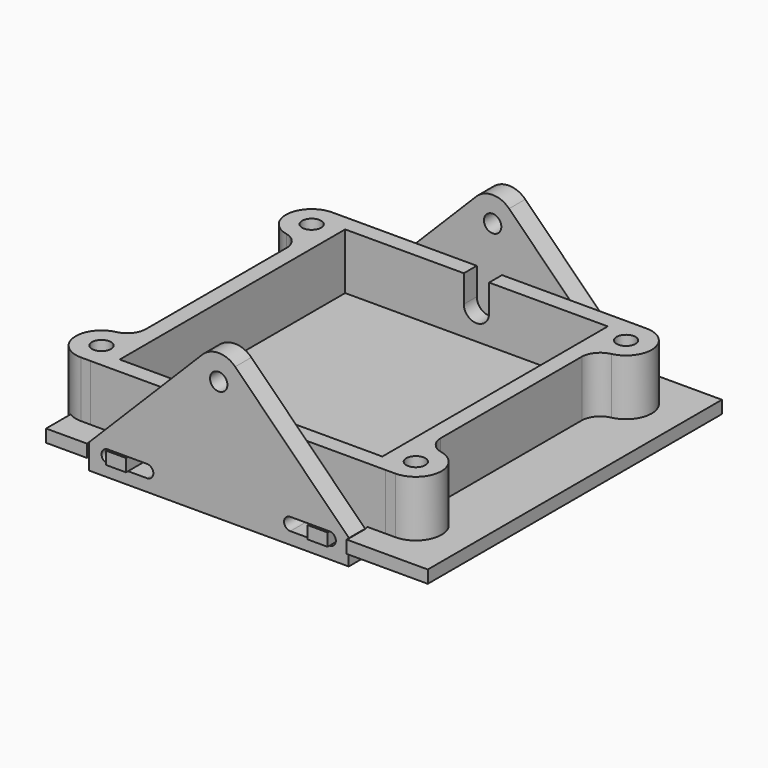
from build123d import *

# Parameters (mm, degrees)
F0_W     = 3.0607
F0_H     = 7.62
F0_W_2   = 2.54
F0_H_2   = 2.8575
F1_DEPTH = 1.5875
F2_R     = 1.0922
F3_DEPTH = 2.54
F5_W     = 33.02
F5_H     = 35.433
F5_R     = 1.1938
F6_DEPTH = 8.636
F8_DEPTH = 42.8635


with BuildPart() as f1:
    # F0 (on Top) → F1 (new body)
    with BuildSketch(Plane.XY):
        with BuildLine():
            Line((-16.32712, 23.114), (-21.4503, 23.114))
            Line((-21.4503, 23.114), (-21.4503, 3.81))
            Line((-21.4503, 3.81), (-21.4503, -3.81))
            Line((-21.4503, -3.81), (-21.4503, -23.114))
            Line((-21.4503, -23.114), (-16.32712, -23.114))
            Line((-16.32712, -23.114), (-16.32712, -20.2565))
            ThreePointArc((-16.32712, -20.2565), (-15.13332, -19.0627), (-13.93952, -20.2565))
            Line((-13.93952, -20.2565), (-11.39952, -20.2565))
            ThreePointArc((-11.39952, -20.2565), (-10.20572, -19.0627), (-9.01192, -20.2565))
            Line((-9.01192, -20.2565), (9.01192, -20.2565))
            ThreePointArc((9.01192, -20.2565), (10.20572, -19.0627), (11.39952, -20.2565))
            Line((11.39952, -20.2565), (13.93952, -20.2565))
            ThreePointArc((13.93952, -20.2565), (15.13332, -19.0627), (16.32712, -20.2565))
            Line((16.32712, -20.2565), (16.32712, -23.114))
            Line((16.32712, -23.114), (21.4503, -23.114))
            Line((21.4503, -23.114), (26.543, -23.114))
            Line((26.543, -23.114), (26.543, 23.114))
            Line((26.543, 23.114), (21.4503, 23.114))
            Line((21.4503, 23.114), (16.32712, 23.114))
            Line((16.32712, 23.114), (16.32712, 20.2565))
            ThreePointArc((16.32712, 20.2565), (15.13332, 19.0627), (13.93952, 20.2565))
            Line((13.93952, 20.2565), (13.93952, 23.114))
            Line((13.93952, 23.114), (11.39952, 23.114))
            Line((11.39952, 23.114), (11.39952, 20.2565))
            ThreePointArc((11.39952, 20.2565), (10.20572, 19.0627), (9.01192, 20.2565))
            Line((9.01192, 20.2565), (-9.01192, 20.2565))
            ThreePointArc((-9.01192, 20.2565), (-10.20572, 19.0627), (-11.39952, 20.2565))
            Line((-11.39952, 20.2565), (-13.93952, 20.2565))
            ThreePointArc((-13.93952, 20.2565), (-15.13332, 19.0627), (-16.32712, 20.2565))
            Line((-16.32712, 20.2565), (-16.32712, 23.114))
        make_face()
        with Locations((-22.98065, 0)):
            Rectangle(F0_W, F0_H)
        with Locations((-12.66952, 21.68525)):
            Rectangle(F0_W_2, F0_H_2)
        with Locations((-12.66952, -21.68525)):
            Rectangle(F0_W_2, F0_H_2)
        with Locations((12.66952, -21.68525)):
            Rectangle(F0_W_2, F0_H_2)
    extrude(amount=F1_DEPTH)


with BuildPart() as f3:
    # F2 (on face) → F3 (new body)
    with BuildSketch(Plane.XZ.offset(20.2565)):
        with BuildLine():
            Line((-11.39952, 1.5875), (-9.01192, 1.5875))
            ThreePointArc((-9.01192, 1.5875), (-8.21817, 0.79375), (-9.01192, 0))
            Line((-9.01192, 0), (9.01192, 0))
            ThreePointArc((9.01192, 0), (8.21817, 0.79375), (9.01192, 1.5875))
            Line((9.01192, 1.5875), (11.39952, 1.5875))
            Line((11.39952, 1.5875), (13.93952, 1.5875))
            ThreePointArc((13.93952, 1.5875), (14.73327, 0.79375), (13.93952, 0))
            Line((13.93952, 0), (16.32712, 0))
            Line((16.32712, 0), (16.3492485881, 0))
            Line((16.3492485881, 0), (16.3747225774, 1.6349537815))
            Line((16.3747225774, 1.6349537815), (2.0716986414, 15.941246014))
            ThreePointArc((2.0716986414, 15.941246014), (0.0017651203, 16.79702), (-2.0656760542, 15.9352422522))
            Line((-2.0656760542, 15.9352422522), (-16.32712, 1.5875))
            Line((-16.32712, 1.5875), (-16.32712, 0))
            Line((-16.32712, 0), (-13.93952, 0))
            ThreePointArc((-13.93952, 0), (-14.73327, 0.79375), (-13.93952, 1.5875))
            Line((-13.93952, 1.5875), (-11.39952, 1.5875))
        make_face()
        with Locations((0, 13.6220204907)):
            Circle(F2_R, mode=Mode.SUBTRACT)
        Polygon((9.01192, 0), (-9.01192, 0), (-11.39952, 0), (-13.93952, 0), (-16.32712, 0), (-16.32712, -1.524), (16.3492485881, -1.524), (16.3492485881, 0), (16.32712, 0), (13.93952, 0), (11.39952, 0), align=None)
    extrude(amount=F3_DEPTH)


with BuildPart() as f4_1:
    # F4: instance of F3
    add(f3.part.mirror(Plane.XZ))


with BuildPart() as f6:
    # F5 (on Top) → F6 (new body)
    with BuildSketch(Plane.XY):
        Polygon((18.542, 19.7485), (-18.542, 19.7485), (-18.542, 11.1380089074), (-18.542, -11.1380089074), (-18.542, -19.7485), (18.542, -19.7485), (18.542, -11.1380089074), (18.542, 11.1380089074), align=None)
        Rectangle(F5_W, F5_H, mode=Mode.SUBTRACT)
        with BuildLine():
            Line((-18.542, 11.1380089074), (-18.542, 19.7485))
            Line((-18.542, 19.7485), (-19.7770799466, 19.7433924169))
            ThreePointArc((-19.7770799466, 19.7433924169), (-22.972674971, 16.8470467627), (-20.4322050252, 13.36184115))
            ThreePointArc((-20.4322050252, 13.36184115), (-19.1077469534, 12.5723683185), (-18.542, 11.1380089074))
        make_face()
        with Locations((-19.76374, 16.51762)):
            Circle(F5_R, mode=Mode.SUBTRACT)
        with BuildLine():
            Line((19.7770799466, 19.7433924169), (18.542, 19.7485))
            Line((18.542, 19.7485), (18.542, 11.1380089074))
            ThreePointArc((18.542, 11.1380089074), (19.1077469534, 12.5723683185), (20.4322050252, 13.36184115))
            ThreePointArc((20.4322050252, 13.36184115), (22.972674971, 16.8470467627), (19.7770799466, 19.7433924169))
        make_face()
        with Locations((19.76374, 16.51762)):
            Circle(F5_R, mode=Mode.SUBTRACT)
        with BuildLine():
            ThreePointArc((20.4322050252, -13.36184115), (19.1077469534, -12.5723683185), (18.542, -11.1380089074))
            Line((18.542, -11.1380089074), (18.542, -19.7485))
            Line((18.542, -19.7485), (19.7770799466, -19.7433924169))
            ThreePointArc((19.7770799466, -19.7433924169), (22.972674971, -16.8470467627), (20.4322050252, -13.36184115))
        make_face()
        with Locations((19.76374, -16.51762)):
            Circle(F5_R, mode=Mode.SUBTRACT)
        with BuildLine():
            Line((-18.542, -19.7485), (-18.542, -11.1380089074))
            ThreePointArc((-18.542, -11.1380089074), (-19.1077469534, -12.5723683185), (-20.4322050252, -13.36184115))
            ThreePointArc((-20.4322050252, -13.36184115), (-22.972674971, -16.8470467627), (-19.7770799466, -19.7433924169))
            Line((-19.7770799466, -19.7433924169), (-18.542, -19.7485))
        make_face()
        with Locations((-19.76374, -16.51762)):
            Circle(F5_R, mode=Mode.SUBTRACT)
    extrude(amount=F6_DEPTH)

    # F7 (on face) → F8 (cut, through all)
    with BuildSketch(Plane.XZ.offset(19.7485)):
        with BuildLine():
            ThreePointArc((1.5875, 5.207), (0, 6.7945), (-1.5875, 5.207))
            ThreePointArc((-1.5875, 5.207), (0, 3.6195), (1.5875, 5.207))
        make_face()
        with BuildLine():
            Line((1.5875, 8.636), (-1.5875, 8.636))
            Line((-1.5875, 8.636), (-1.5875, 5.207))
            ThreePointArc((-1.5875, 5.207), (0, 6.7945), (1.5875, 5.207))
            Line((1.5875, 5.207), (1.5875, 8.636))
        make_face()
    extrude(amount=-F8_DEPTH, mode=Mode.SUBTRACT)


solid = Compound([f1.part, f3.part, f4_1.part, f6.part])
